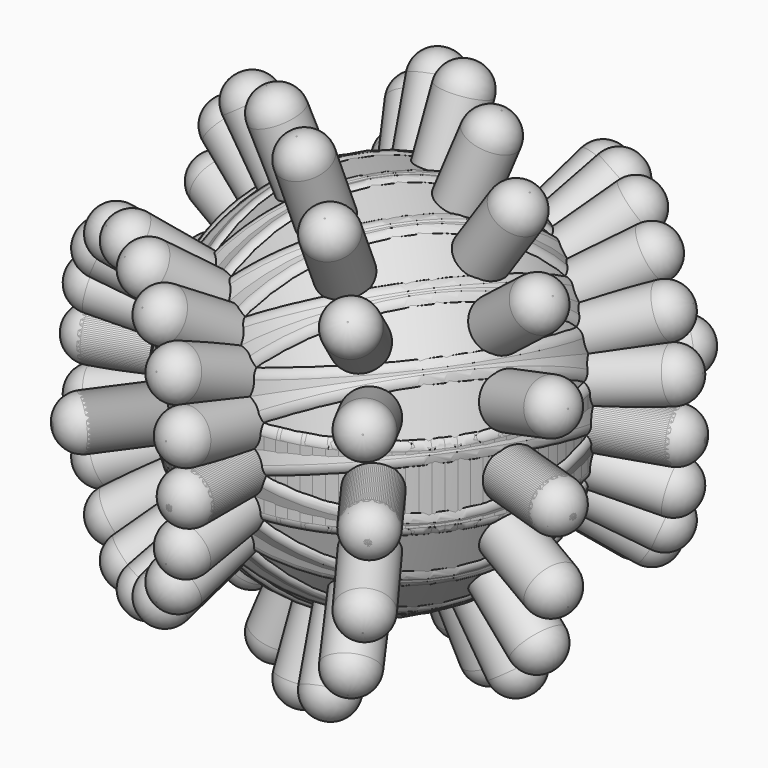
from build123d import *

# Parameters (mm, degrees)
F0_R     = 22.3611079821
F0_R_2   = 12.9291166365
F1_DEPTH = 10.922
F2_R     = 1.27
F4_START = -21.336
F3_R     = 3.1244173249
F4_DEPTH = 11.938
F5_R     = 3.048
F6_COUNT = 10
F7_COUNT = 10
F7_ANGLE = 180


with BuildPart() as f1:
    # F0 (on Top) → F1 (new body)
    with BuildSketch(Plane.XY):
        Circle(F0_R)
        Circle(F0_R_2, mode=Mode.SUBTRACT)
    extrude(amount=-F1_DEPTH)

    # F2
    f2_edges = [f1.edges().sort_by_distance(p)[0] for p in [
        (-22.361108, 0, 0),
        (-22.361108, 0, -10.922),
    ]]
    fillet(f2_edges, radius=F2_R)


with BuildPart() as f4:
    # F3 (on Front) → F4 (new body)
    with BuildSketch(Plane.XZ.offset(F4_START)):
        with Locations((0, -5.461)):
            Circle(F3_R)
    extrude(amount=-F4_DEPTH)

    # F5
    f5_edges = [f4.edges().sort_by_distance(p)[0] for p in [
        (-3.124417, 33.274, -5.461),
    ]]
    fillet(f5_edges, radius=F5_R)


with BuildPart() as f6_1:
    # F6: instance of F4
    add(f4.part.rotate(Axis((0, 0, 0), (0, 0, 1)), 1 * 360 / F6_COUNT))


with BuildPart() as f6_2:
    # F6: instance of F4
    add(f4.part.rotate(Axis((0, 0, 0), (0, 0, 1)), 2 * 360 / F6_COUNT))


with BuildPart() as f6_3:
    # F6: instance of F4
    add(f4.part.rotate(Axis((0, 0, 0), (0, 0, 1)), 3 * 360 / F6_COUNT))


with BuildPart() as f6_4:
    # F6: instance of F4
    add(f4.part.rotate(Axis((0, 0, 0), (0, 0, 1)), 4 * 360 / F6_COUNT))


with BuildPart() as f6_5:
    # F6: instance of F4
    add(f4.part.rotate(Axis((0, 0, 0), (0, 0, 1)), 5 * 360 / F6_COUNT))


with BuildPart() as f6_6:
    # F6: instance of F4
    add(f4.part.rotate(Axis((0, 0, 0), (0, 0, 1)), 6 * 360 / F6_COUNT))


with BuildPart() as f6_7:
    # F6: instance of F4
    add(f4.part.rotate(Axis((0, 0, 0), (0, 0, 1)), 7 * 360 / F6_COUNT))


with BuildPart() as f6_8:
    # F6: instance of F4
    add(f4.part.rotate(Axis((0, 0, 0), (0, 0, 1)), 8 * 360 / F6_COUNT))


with BuildPart() as f6_9:
    # F6: instance of F4
    add(f4.part.rotate(Axis((0, 0, 0), (0, 0, 1)), 9 * 360 / F6_COUNT))


with BuildPart() as f7_1:
    # F7: instance of F1
    add(f1.part.rotate(Axis((12.5409861429, 17.261186592, -5.461), (-0.5877852523, -0.8090169944, 0)), 1 * F7_ANGLE / (F7_COUNT - 1)))


with BuildPart() as f7_2:
    # F7: instance of F1
    add(f1.part.rotate(Axis((12.5409861429, 17.261186592, -5.461), (-0.5877852523, -0.8090169944, 0)), 2 * F7_ANGLE / (F7_COUNT - 1)))


with BuildPart() as f7_3:
    # F7: instance of F1
    add(f1.part.rotate(Axis((12.5409861429, 17.261186592, -5.461), (-0.5877852523, -0.8090169944, 0)), 3 * F7_ANGLE / (F7_COUNT - 1)))


with BuildPart() as f7_4:
    # F7: instance of F1
    add(f1.part.rotate(Axis((12.5409861429, 17.261186592, -5.461), (-0.5877852523, -0.8090169944, 0)), 4 * F7_ANGLE / (F7_COUNT - 1)))


with BuildPart() as f7_5:
    # F7: instance of F1
    add(f1.part.rotate(Axis((12.5409861429, 17.261186592, -5.461), (-0.5877852523, -0.8090169944, 0)), 5 * F7_ANGLE / (F7_COUNT - 1)))


with BuildPart() as f7_6:
    # F7: instance of F1
    add(f1.part.rotate(Axis((12.5409861429, 17.261186592, -5.461), (-0.5877852523, -0.8090169944, 0)), 6 * F7_ANGLE / (F7_COUNT - 1)))


with BuildPart() as f7_7:
    # F7: instance of F1
    add(f1.part.rotate(Axis((12.5409861429, 17.261186592, -5.461), (-0.5877852523, -0.8090169944, 0)), 7 * F7_ANGLE / (F7_COUNT - 1)))


with BuildPart() as f7_8:
    # F7: instance of F1
    add(f1.part.rotate(Axis((12.5409861429, 17.261186592, -5.461), (-0.5877852523, -0.8090169944, 0)), 8 * F7_ANGLE / (F7_COUNT - 1)))


with BuildPart() as f7_9:
    # F7: instance of F1
    add(f1.part.rotate(Axis((12.5409861429, 17.261186592, -5.461), (-0.5877852523, -0.8090169944, 0)), 9 * F7_ANGLE / (F7_COUNT - 1)))


with BuildPart() as f7_10:
    # F7: instance of F6_8
    add(f6_8.part.rotate(Axis((12.5409861429, 17.261186592, -5.461), (-0.5877852523, -0.8090169944, 0)), 1 * F7_ANGLE / (F7_COUNT - 1)))


with BuildPart() as f7_11:
    # F7: instance of F6_8
    add(f6_8.part.rotate(Axis((12.5409861429, 17.261186592, -5.461), (-0.5877852523, -0.8090169944, 0)), 2 * F7_ANGLE / (F7_COUNT - 1)))


with BuildPart() as f7_12:
    # F7: instance of F6_8
    add(f6_8.part.rotate(Axis((12.5409861429, 17.261186592, -5.461), (-0.5877852523, -0.8090169944, 0)), 3 * F7_ANGLE / (F7_COUNT - 1)))


with BuildPart() as f7_13:
    # F7: instance of F6_8
    add(f6_8.part.rotate(Axis((12.5409861429, 17.261186592, -5.461), (-0.5877852523, -0.8090169944, 0)), 4 * F7_ANGLE / (F7_COUNT - 1)))


with BuildPart() as f7_14:
    # F7: instance of F6_8
    add(f6_8.part.rotate(Axis((12.5409861429, 17.261186592, -5.461), (-0.5877852523, -0.8090169944, 0)), 5 * F7_ANGLE / (F7_COUNT - 1)))


with BuildPart() as f7_15:
    # F7: instance of F6_8
    add(f6_8.part.rotate(Axis((12.5409861429, 17.261186592, -5.461), (-0.5877852523, -0.8090169944, 0)), 6 * F7_ANGLE / (F7_COUNT - 1)))


with BuildPart() as f7_16:
    # F7: instance of F6_8
    add(f6_8.part.rotate(Axis((12.5409861429, 17.261186592, -5.461), (-0.5877852523, -0.8090169944, 0)), 7 * F7_ANGLE / (F7_COUNT - 1)))


with BuildPart() as f7_17:
    # F7: instance of F6_8
    add(f6_8.part.rotate(Axis((12.5409861429, 17.261186592, -5.461), (-0.5877852523, -0.8090169944, 0)), 8 * F7_ANGLE / (F7_COUNT - 1)))


with BuildPart() as f7_18:
    # F7: instance of F6_8
    add(f6_8.part.rotate(Axis((12.5409861429, 17.261186592, -5.461), (-0.5877852523, -0.8090169944, 0)), 9 * F7_ANGLE / (F7_COUNT - 1)))


with BuildPart() as f7_19:
    # F7: instance of F6_7
    add(f6_7.part.rotate(Axis((12.5409861429, 17.261186592, -5.461), (-0.5877852523, -0.8090169944, 0)), 1 * F7_ANGLE / (F7_COUNT - 1)))


with BuildPart() as f7_20:
    # F7: instance of F6_7
    add(f6_7.part.rotate(Axis((12.5409861429, 17.261186592, -5.461), (-0.5877852523, -0.8090169944, 0)), 2 * F7_ANGLE / (F7_COUNT - 1)))


with BuildPart() as f7_21:
    # F7: instance of F6_7
    add(f6_7.part.rotate(Axis((12.5409861429, 17.261186592, -5.461), (-0.5877852523, -0.8090169944, 0)), 3 * F7_ANGLE / (F7_COUNT - 1)))


with BuildPart() as f7_22:
    # F7: instance of F6_7
    add(f6_7.part.rotate(Axis((12.5409861429, 17.261186592, -5.461), (-0.5877852523, -0.8090169944, 0)), 4 * F7_ANGLE / (F7_COUNT - 1)))


with BuildPart() as f7_23:
    # F7: instance of F6_7
    add(f6_7.part.rotate(Axis((12.5409861429, 17.261186592, -5.461), (-0.5877852523, -0.8090169944, 0)), 5 * F7_ANGLE / (F7_COUNT - 1)))


with BuildPart() as f7_24:
    # F7: instance of F6_7
    add(f6_7.part.rotate(Axis((12.5409861429, 17.261186592, -5.461), (-0.5877852523, -0.8090169944, 0)), 6 * F7_ANGLE / (F7_COUNT - 1)))


with BuildPart() as f7_25:
    # F7: instance of F6_7
    add(f6_7.part.rotate(Axis((12.5409861429, 17.261186592, -5.461), (-0.5877852523, -0.8090169944, 0)), 7 * F7_ANGLE / (F7_COUNT - 1)))


with BuildPart() as f7_26:
    # F7: instance of F6_7
    add(f6_7.part.rotate(Axis((12.5409861429, 17.261186592, -5.461), (-0.5877852523, -0.8090169944, 0)), 8 * F7_ANGLE / (F7_COUNT - 1)))


with BuildPart() as f7_27:
    # F7: instance of F6_7
    add(f6_7.part.rotate(Axis((12.5409861429, 17.261186592, -5.461), (-0.5877852523, -0.8090169944, 0)), 9 * F7_ANGLE / (F7_COUNT - 1)))


with BuildPart() as f7_28:
    # F7: instance of F6_6
    add(f6_6.part.rotate(Axis((12.5409861429, 17.261186592, -5.461), (-0.5877852523, -0.8090169944, 0)), 1 * F7_ANGLE / (F7_COUNT - 1)))


with BuildPart() as f7_29:
    # F7: instance of F6_6
    add(f6_6.part.rotate(Axis((12.5409861429, 17.261186592, -5.461), (-0.5877852523, -0.8090169944, 0)), 2 * F7_ANGLE / (F7_COUNT - 1)))


with BuildPart() as f7_30:
    # F7: instance of F6_6
    add(f6_6.part.rotate(Axis((12.5409861429, 17.261186592, -5.461), (-0.5877852523, -0.8090169944, 0)), 3 * F7_ANGLE / (F7_COUNT - 1)))


with BuildPart() as f7_31:
    # F7: instance of F6_6
    add(f6_6.part.rotate(Axis((12.5409861429, 17.261186592, -5.461), (-0.5877852523, -0.8090169944, 0)), 4 * F7_ANGLE / (F7_COUNT - 1)))


with BuildPart() as f7_32:
    # F7: instance of F6_6
    add(f6_6.part.rotate(Axis((12.5409861429, 17.261186592, -5.461), (-0.5877852523, -0.8090169944, 0)), 5 * F7_ANGLE / (F7_COUNT - 1)))


with BuildPart() as f7_33:
    # F7: instance of F6_6
    add(f6_6.part.rotate(Axis((12.5409861429, 17.261186592, -5.461), (-0.5877852523, -0.8090169944, 0)), 6 * F7_ANGLE / (F7_COUNT - 1)))


with BuildPart() as f7_34:
    # F7: instance of F6_6
    add(f6_6.part.rotate(Axis((12.5409861429, 17.261186592, -5.461), (-0.5877852523, -0.8090169944, 0)), 7 * F7_ANGLE / (F7_COUNT - 1)))


with BuildPart() as f7_35:
    # F7: instance of F6_6
    add(f6_6.part.rotate(Axis((12.5409861429, 17.261186592, -5.461), (-0.5877852523, -0.8090169944, 0)), 8 * F7_ANGLE / (F7_COUNT - 1)))


with BuildPart() as f7_36:
    # F7: instance of F6_6
    add(f6_6.part.rotate(Axis((12.5409861429, 17.261186592, -5.461), (-0.5877852523, -0.8090169944, 0)), 9 * F7_ANGLE / (F7_COUNT - 1)))


with BuildPart() as f7_37:
    # F7: instance of F6_5
    add(f6_5.part.rotate(Axis((12.5409861429, 17.261186592, -5.461), (-0.5877852523, -0.8090169944, 0)), 1 * F7_ANGLE / (F7_COUNT - 1)))


with BuildPart() as f7_38:
    # F7: instance of F6_5
    add(f6_5.part.rotate(Axis((12.5409861429, 17.261186592, -5.461), (-0.5877852523, -0.8090169944, 0)), 2 * F7_ANGLE / (F7_COUNT - 1)))


with BuildPart() as f7_39:
    # F7: instance of F6_5
    add(f6_5.part.rotate(Axis((12.5409861429, 17.261186592, -5.461), (-0.5877852523, -0.8090169944, 0)), 3 * F7_ANGLE / (F7_COUNT - 1)))


with BuildPart() as f7_40:
    # F7: instance of F6_5
    add(f6_5.part.rotate(Axis((12.5409861429, 17.261186592, -5.461), (-0.5877852523, -0.8090169944, 0)), 4 * F7_ANGLE / (F7_COUNT - 1)))


with BuildPart() as f7_41:
    # F7: instance of F6_5
    add(f6_5.part.rotate(Axis((12.5409861429, 17.261186592, -5.461), (-0.5877852523, -0.8090169944, 0)), 5 * F7_ANGLE / (F7_COUNT - 1)))


with BuildPart() as f7_42:
    # F7: instance of F6_5
    add(f6_5.part.rotate(Axis((12.5409861429, 17.261186592, -5.461), (-0.5877852523, -0.8090169944, 0)), 6 * F7_ANGLE / (F7_COUNT - 1)))


with BuildPart() as f7_43:
    # F7: instance of F6_5
    add(f6_5.part.rotate(Axis((12.5409861429, 17.261186592, -5.461), (-0.5877852523, -0.8090169944, 0)), 7 * F7_ANGLE / (F7_COUNT - 1)))


with BuildPart() as f7_44:
    # F7: instance of F6_5
    add(f6_5.part.rotate(Axis((12.5409861429, 17.261186592, -5.461), (-0.5877852523, -0.8090169944, 0)), 8 * F7_ANGLE / (F7_COUNT - 1)))


with BuildPart() as f7_45:
    # F7: instance of F6_5
    add(f6_5.part.rotate(Axis((12.5409861429, 17.261186592, -5.461), (-0.5877852523, -0.8090169944, 0)), 9 * F7_ANGLE / (F7_COUNT - 1)))


with BuildPart() as f7_46:
    # F7: instance of F6_4
    add(f6_4.part.rotate(Axis((12.5409861429, 17.261186592, -5.461), (-0.5877852523, -0.8090169944, 0)), 1 * F7_ANGLE / (F7_COUNT - 1)))


with BuildPart() as f7_47:
    # F7: instance of F6_4
    add(f6_4.part.rotate(Axis((12.5409861429, 17.261186592, -5.461), (-0.5877852523, -0.8090169944, 0)), 2 * F7_ANGLE / (F7_COUNT - 1)))


with BuildPart() as f7_48:
    # F7: instance of F6_4
    add(f6_4.part.rotate(Axis((12.5409861429, 17.261186592, -5.461), (-0.5877852523, -0.8090169944, 0)), 3 * F7_ANGLE / (F7_COUNT - 1)))


with BuildPart() as f7_49:
    # F7: instance of F6_4
    add(f6_4.part.rotate(Axis((12.5409861429, 17.261186592, -5.461), (-0.5877852523, -0.8090169944, 0)), 4 * F7_ANGLE / (F7_COUNT - 1)))


with BuildPart() as f7_50:
    # F7: instance of F6_4
    add(f6_4.part.rotate(Axis((12.5409861429, 17.261186592, -5.461), (-0.5877852523, -0.8090169944, 0)), 5 * F7_ANGLE / (F7_COUNT - 1)))


with BuildPart() as f7_51:
    # F7: instance of F6_4
    add(f6_4.part.rotate(Axis((12.5409861429, 17.261186592, -5.461), (-0.5877852523, -0.8090169944, 0)), 6 * F7_ANGLE / (F7_COUNT - 1)))


with BuildPart() as f7_52:
    # F7: instance of F6_4
    add(f6_4.part.rotate(Axis((12.5409861429, 17.261186592, -5.461), (-0.5877852523, -0.8090169944, 0)), 7 * F7_ANGLE / (F7_COUNT - 1)))


with BuildPart() as f7_53:
    # F7: instance of F6_4
    add(f6_4.part.rotate(Axis((12.5409861429, 17.261186592, -5.461), (-0.5877852523, -0.8090169944, 0)), 8 * F7_ANGLE / (F7_COUNT - 1)))


with BuildPart() as f7_54:
    # F7: instance of F6_4
    add(f6_4.part.rotate(Axis((12.5409861429, 17.261186592, -5.461), (-0.5877852523, -0.8090169944, 0)), 9 * F7_ANGLE / (F7_COUNT - 1)))


with BuildPart() as f7_55:
    # F7: instance of F6_3
    add(f6_3.part.rotate(Axis((12.5409861429, 17.261186592, -5.461), (-0.5877852523, -0.8090169944, 0)), 1 * F7_ANGLE / (F7_COUNT - 1)))


with BuildPart() as f7_56:
    # F7: instance of F6_3
    add(f6_3.part.rotate(Axis((12.5409861429, 17.261186592, -5.461), (-0.5877852523, -0.8090169944, 0)), 2 * F7_ANGLE / (F7_COUNT - 1)))


with BuildPart() as f7_57:
    # F7: instance of F6_3
    add(f6_3.part.rotate(Axis((12.5409861429, 17.261186592, -5.461), (-0.5877852523, -0.8090169944, 0)), 3 * F7_ANGLE / (F7_COUNT - 1)))


with BuildPart() as f7_58:
    # F7: instance of F6_3
    add(f6_3.part.rotate(Axis((12.5409861429, 17.261186592, -5.461), (-0.5877852523, -0.8090169944, 0)), 4 * F7_ANGLE / (F7_COUNT - 1)))


with BuildPart() as f7_59:
    # F7: instance of F6_3
    add(f6_3.part.rotate(Axis((12.5409861429, 17.261186592, -5.461), (-0.5877852523, -0.8090169944, 0)), 5 * F7_ANGLE / (F7_COUNT - 1)))


with BuildPart() as f7_60:
    # F7: instance of F6_3
    add(f6_3.part.rotate(Axis((12.5409861429, 17.261186592, -5.461), (-0.5877852523, -0.8090169944, 0)), 6 * F7_ANGLE / (F7_COUNT - 1)))


with BuildPart() as f7_61:
    # F7: instance of F6_3
    add(f6_3.part.rotate(Axis((12.5409861429, 17.261186592, -5.461), (-0.5877852523, -0.8090169944, 0)), 7 * F7_ANGLE / (F7_COUNT - 1)))


with BuildPart() as f7_62:
    # F7: instance of F6_3
    add(f6_3.part.rotate(Axis((12.5409861429, 17.261186592, -5.461), (-0.5877852523, -0.8090169944, 0)), 8 * F7_ANGLE / (F7_COUNT - 1)))


with BuildPart() as f7_63:
    # F7: instance of F6_3
    add(f6_3.part.rotate(Axis((12.5409861429, 17.261186592, -5.461), (-0.5877852523, -0.8090169944, 0)), 9 * F7_ANGLE / (F7_COUNT - 1)))


with BuildPart() as f7_64:
    # F7: instance of F6_2
    add(f6_2.part.rotate(Axis((12.5409861429, 17.261186592, -5.461), (-0.5877852523, -0.8090169944, 0)), 1 * F7_ANGLE / (F7_COUNT - 1)))


with BuildPart() as f7_65:
    # F7: instance of F6_2
    add(f6_2.part.rotate(Axis((12.5409861429, 17.261186592, -5.461), (-0.5877852523, -0.8090169944, 0)), 2 * F7_ANGLE / (F7_COUNT - 1)))


with BuildPart() as f7_66:
    # F7: instance of F6_2
    add(f6_2.part.rotate(Axis((12.5409861429, 17.261186592, -5.461), (-0.5877852523, -0.8090169944, 0)), 3 * F7_ANGLE / (F7_COUNT - 1)))


with BuildPart() as f7_67:
    # F7: instance of F6_2
    add(f6_2.part.rotate(Axis((12.5409861429, 17.261186592, -5.461), (-0.5877852523, -0.8090169944, 0)), 4 * F7_ANGLE / (F7_COUNT - 1)))


with BuildPart() as f7_68:
    # F7: instance of F6_2
    add(f6_2.part.rotate(Axis((12.5409861429, 17.261186592, -5.461), (-0.5877852523, -0.8090169944, 0)), 5 * F7_ANGLE / (F7_COUNT - 1)))


with BuildPart() as f7_69:
    # F7: instance of F6_2
    add(f6_2.part.rotate(Axis((12.5409861429, 17.261186592, -5.461), (-0.5877852523, -0.8090169944, 0)), 6 * F7_ANGLE / (F7_COUNT - 1)))


with BuildPart() as f7_70:
    # F7: instance of F6_2
    add(f6_2.part.rotate(Axis((12.5409861429, 17.261186592, -5.461), (-0.5877852523, -0.8090169944, 0)), 7 * F7_ANGLE / (F7_COUNT - 1)))


with BuildPart() as f7_71:
    # F7: instance of F6_2
    add(f6_2.part.rotate(Axis((12.5409861429, 17.261186592, -5.461), (-0.5877852523, -0.8090169944, 0)), 8 * F7_ANGLE / (F7_COUNT - 1)))


with BuildPart() as f7_72:
    # F7: instance of F6_2
    add(f6_2.part.rotate(Axis((12.5409861429, 17.261186592, -5.461), (-0.5877852523, -0.8090169944, 0)), 9 * F7_ANGLE / (F7_COUNT - 1)))


with BuildPart() as f7_73:
    # F7: instance of F6_1
    add(f6_1.part.rotate(Axis((12.5409861429, 17.261186592, -5.461), (-0.5877852523, -0.8090169944, 0)), 1 * F7_ANGLE / (F7_COUNT - 1)))


with BuildPart() as f7_74:
    # F7: instance of F6_1
    add(f6_1.part.rotate(Axis((12.5409861429, 17.261186592, -5.461), (-0.5877852523, -0.8090169944, 0)), 2 * F7_ANGLE / (F7_COUNT - 1)))


with BuildPart() as f7_75:
    # F7: instance of F6_1
    add(f6_1.part.rotate(Axis((12.5409861429, 17.261186592, -5.461), (-0.5877852523, -0.8090169944, 0)), 3 * F7_ANGLE / (F7_COUNT - 1)))


with BuildPart() as f7_76:
    # F7: instance of F6_1
    add(f6_1.part.rotate(Axis((12.5409861429, 17.261186592, -5.461), (-0.5877852523, -0.8090169944, 0)), 4 * F7_ANGLE / (F7_COUNT - 1)))


with BuildPart() as f7_77:
    # F7: instance of F6_1
    add(f6_1.part.rotate(Axis((12.5409861429, 17.261186592, -5.461), (-0.5877852523, -0.8090169944, 0)), 5 * F7_ANGLE / (F7_COUNT - 1)))


with BuildPart() as f7_78:
    # F7: instance of F6_1
    add(f6_1.part.rotate(Axis((12.5409861429, 17.261186592, -5.461), (-0.5877852523, -0.8090169944, 0)), 6 * F7_ANGLE / (F7_COUNT - 1)))


with BuildPart() as f7_79:
    # F7: instance of F6_1
    add(f6_1.part.rotate(Axis((12.5409861429, 17.261186592, -5.461), (-0.5877852523, -0.8090169944, 0)), 7 * F7_ANGLE / (F7_COUNT - 1)))


with BuildPart() as f7_80:
    # F7: instance of F6_1
    add(f6_1.part.rotate(Axis((12.5409861429, 17.261186592, -5.461), (-0.5877852523, -0.8090169944, 0)), 8 * F7_ANGLE / (F7_COUNT - 1)))


with BuildPart() as f7_81:
    # F7: instance of F6_1
    add(f6_1.part.rotate(Axis((12.5409861429, 17.261186592, -5.461), (-0.5877852523, -0.8090169944, 0)), 9 * F7_ANGLE / (F7_COUNT - 1)))


with BuildPart() as f7_82:
    # F7: instance of F4
    add(f4.part.rotate(Axis((12.5409861429, 17.261186592, -5.461), (-0.5877852523, -0.8090169944, 0)), 1 * F7_ANGLE / (F7_COUNT - 1)))


with BuildPart() as f7_83:
    # F7: instance of F4
    add(f4.part.rotate(Axis((12.5409861429, 17.261186592, -5.461), (-0.5877852523, -0.8090169944, 0)), 2 * F7_ANGLE / (F7_COUNT - 1)))


with BuildPart() as f7_84:
    # F7: instance of F4
    add(f4.part.rotate(Axis((12.5409861429, 17.261186592, -5.461), (-0.5877852523, -0.8090169944, 0)), 3 * F7_ANGLE / (F7_COUNT - 1)))


with BuildPart() as f7_85:
    # F7: instance of F4
    add(f4.part.rotate(Axis((12.5409861429, 17.261186592, -5.461), (-0.5877852523, -0.8090169944, 0)), 4 * F7_ANGLE / (F7_COUNT - 1)))


with BuildPart() as f7_86:
    # F7: instance of F4
    add(f4.part.rotate(Axis((12.5409861429, 17.261186592, -5.461), (-0.5877852523, -0.8090169944, 0)), 5 * F7_ANGLE / (F7_COUNT - 1)))


with BuildPart() as f7_87:
    # F7: instance of F4
    add(f4.part.rotate(Axis((12.5409861429, 17.261186592, -5.461), (-0.5877852523, -0.8090169944, 0)), 6 * F7_ANGLE / (F7_COUNT - 1)))


with BuildPart() as f7_88:
    # F7: instance of F4
    add(f4.part.rotate(Axis((12.5409861429, 17.261186592, -5.461), (-0.5877852523, -0.8090169944, 0)), 7 * F7_ANGLE / (F7_COUNT - 1)))


with BuildPart() as f7_89:
    # F7: instance of F4
    add(f4.part.rotate(Axis((12.5409861429, 17.261186592, -5.461), (-0.5877852523, -0.8090169944, 0)), 8 * F7_ANGLE / (F7_COUNT - 1)))


with BuildPart() as f7_90:
    # F7: instance of F4
    add(f4.part.rotate(Axis((12.5409861429, 17.261186592, -5.461), (-0.5877852523, -0.8090169944, 0)), 9 * F7_ANGLE / (F7_COUNT - 1)))


solid = Compound([f1.part, f4.part, f6_1.part, f6_2.part, f6_3.part, f6_4.part, f6_5.part, f6_6.part, f6_7.part, f6_8.part, f6_9.part, f7_1.part, f7_2.part, f7_3.part, f7_4.part, f7_5.part, f7_6.part, f7_7.part, f7_8.part, f7_9.part, f7_10.part, f7_11.part, f7_12.part, f7_13.part, f7_14.part, f7_15.part, f7_16.part, f7_17.part, f7_18.part, f7_19.part, f7_20.part, f7_21.part, f7_22.part, f7_23.part, f7_24.part, f7_25.part, f7_26.part, f7_27.part, f7_28.part, f7_29.part, f7_30.part, f7_31.part, f7_32.part, f7_33.part, f7_34.part, f7_35.part, f7_36.part, f7_37.part, f7_38.part, f7_39.part, f7_40.part, f7_41.part, f7_42.part, f7_43.part, f7_44.part, f7_45.part, f7_46.part, f7_47.part, f7_48.part, f7_49.part, f7_50.part, f7_51.part, f7_52.part, f7_53.part, f7_54.part, f7_55.part, f7_56.part, f7_57.part, f7_58.part, f7_59.part, f7_60.part, f7_61.part, f7_62.part, f7_63.part, f7_64.part, f7_65.part, f7_66.part, f7_67.part, f7_68.part, f7_69.part, f7_70.part, f7_71.part, f7_72.part, f7_73.part, f7_74.part, f7_75.part, f7_76.part, f7_77.part, f7_78.part, f7_79.part, f7_80.part, f7_81.part, f7_82.part, f7_83.part, f7_84.part, f7_85.part, f7_86.part, f7_87.part, f7_88.part, f7_89.part, f7_90.part])
